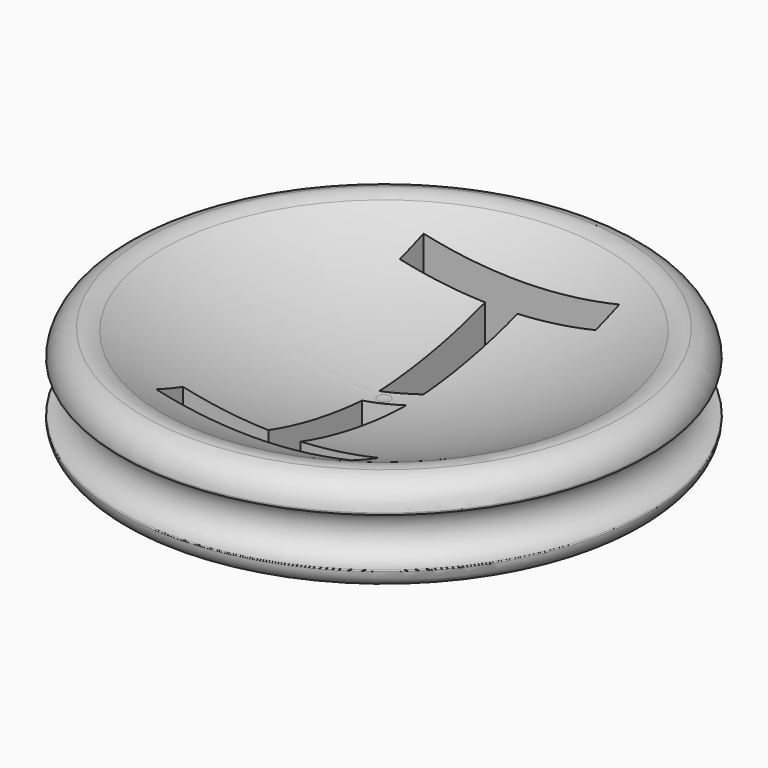
from build123d import *

# Parameters (mm, degrees)
F3_DEPTH = 25


# Not quite as in the source:
# - a feature names something its author has since deleted; it is built from what else it names


with BuildPart() as f1:
    # F0 (on Front) → F1 (revolve)
    with BuildSketch(Plane.XZ):
        with BuildLine():
            ThreePointArc((-27.4979237057, -10.8468195568), (-26.8816261832, -12.2017772322), (-25.5, -12.7557104668))
            Line((-25.5, -12.7557104668), (-25, -12.7557104668))
            Line((-25, -12.7557104668), (-25, -2.7763174613))
            ThreePointArc((-25, -2.7763174613), (-26.6987851099, -3.6934399021), (-27.4870326809, -5.4557254034))
            ThreePointArc((-27.4870326809, -5.4557254034), (-27.4342006293, -5.6429676648), (-27.2702117083, -5.7476506334))
            ThreePointArc((-27.2702117083, -5.7476506334), (-25.02015453, -8.3174880746), (-27.4147150934, -10.7532428834))
            ThreePointArc((-27.4147150934, -10.7532428834), (-27.4742431694, -10.784093359), (-27.4979237057, -10.8468195568))
        make_face()
        with BuildLine():
            Line((-25, -2.7763174613), (-25, -12.7557104668))
            Line((-25, -12.7557104668), (0.1083903732, -12.7557104668))
            Line((0.1083903732, -12.7557104668), (0.1083903732, -9.7607430522))
            Line((0.1083903732, -9.7607430522), (0.1083903732, -9.2934911311))
            Line((0.1083903732, -9.2934911311), (-0.5557517075, -9.2580601338))
            ThreePointArc((-0.5557517075, -9.2580601338), (-12.1652391069, -7.3795693077), (-23.1099525663, -3.075829916))
            ThreePointArc((-23.1099525663, -3.075829916), (-24.0304544365, -2.7713306969), (-25, -2.7763174613))
        make_face()
    revolve(axis=Axis((0.1083903732, 0, -5.038301622), (0, 0, -1)))

    # F2 (on Top) → F3 (cut)
    with BuildSketch(Plane.XY):
        Polygon((2.4412334897, 0), (-0.9498652071, -1.5360242687), (-0.9498652071, -13.7900933623), (-9.8661333323, -13.7900933623), (-9.8661333323, -17.3187889159), (10.6026176363, -17.3187889159), (10.6026176363, -13.7900933623), (2.4412334897, -13.7900933623), align=None)
        Polygon((-0.9498652071, 14.5563995466), (-0.9498652071, 1.5588715905), (-0.9498652071, 0.7185048307), (2.4412334897, 2.2559929639), (2.4412334897, 3.1213716138), (2.4412334897, 14.5563995466), (10.6026176363, 14.5563995466), (10.6026176363, 17.6499914378), (-9.8661333323, 17.6499914378), (-9.8661333323, 14.5563995466), align=None)
    extrude(amount=-F3_DEPTH, mode=Mode.SUBTRACT)


solid = f1.part
